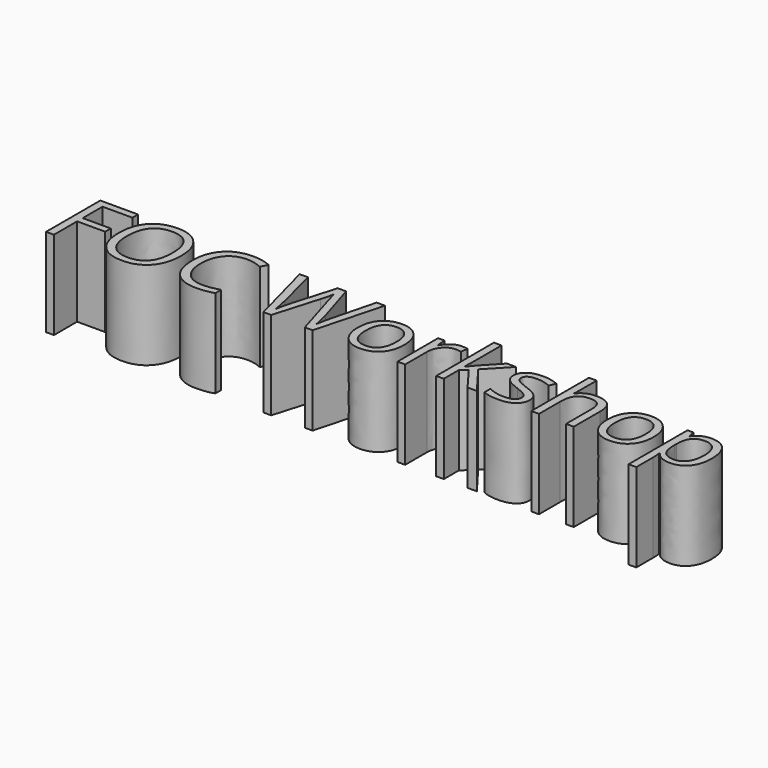
from build123d import *

# Parameters (mm, degrees)
F0_TEXT_SIZE = 27.2690008084
F1_DEPTH     = 25.4


# Not quite as in the source:
# - Text() gives the source's letters only with a copy of the font that has no kerning and outlines rounded to 1/6400 em; it was checked with that copy


with BuildPart() as f1:
    # F0 (on Top) → F1 (new body)
    with BuildSketch(Plane.XY):
        with Locations((-68.5434192419, 83.1538066268)):
            Text('FOC Workshop', F0_TEXT_SIZE, font='Open Sans', text_align=(TextAlign.LEFT, TextAlign.BOTTOM))
    extrude(amount=F1_DEPTH)


solid = f1.part
